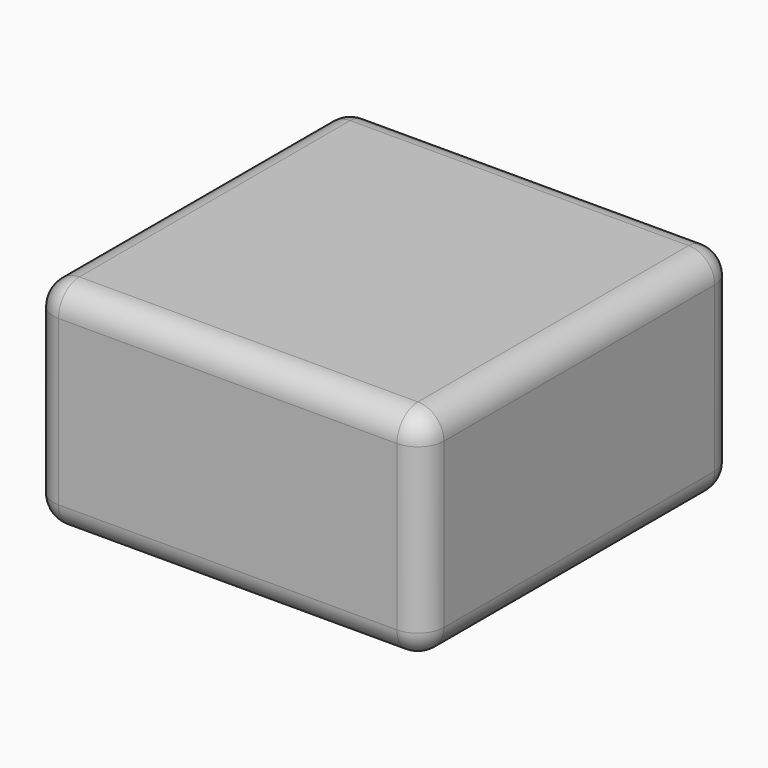
from build123d import *

# Parameters (mm, degrees)
F0_W         = 76.2
F0_H         = 76.2
F0_W_2       = 3.4224579499
F0_H_2       = 7.5862997554
F1_DEPTH     = 42.164
F2_R         = 5.08
F3_T1_DEPTH  = 32.004
F3_S5_W      = 5.08
F3_S5_H      = 5.08
F3_T6_DEPTH  = 5.08
F3_S11_W     = 5.08
F3_S11_H     = 5.08
F3_T12_DEPTH = 5.08


# Not quite as in the source:
# - a fillet or chamfer that OpenCascade refuses, or shapes differently, is made with other operations: its cross-section is extruded or revolved along the edge and cut away or added


with BuildPart() as f1:
    # F0 (on Top) → F1 (new body)
    with BuildSketch(Plane.XY):
        with Locations((-41.3324069232, -13.9183843632)):
            Rectangle(F0_W, F0_H)
        with Locations((-63.0685785115, -38.5174307738)):
            Rectangle(F0_W_2, F0_H_2, mode=Mode.SUBTRACT)
        with Locations((-63.0685785115, -38.5174307738)):
            Rectangle(F0_W_2, F0_H_2)
    extrude(amount=F1_DEPTH)

    # F2
    f2_edges = [f1.edges().sort_by_distance(p)[0] for p in [
        (-41.332407, -52.018384, 0),
        (-3.232407, -13.918384, 0),
        (-41.332407, 24.181616, 0),
        (-79.432407, -13.918384, 0),
        (-79.432407, 24.181616, 21.082),
        (-79.432407, -52.018384, 21.082),
        (-79.432407, -13.918384, 42.164),
        (-41.332407, -52.018384, 42.164),
        (-3.232407, -13.918384, 42.164),
        (-41.332407, 24.181616, 42.164),
        (-3.232407, 24.181616, 21.082),
    ]]
    fillet(f2_edges, radius=F2_R)

    # F3: fillet of radius 5.08 on 1 edges, made by hand

    # F3_s2 → F3_t1 (cut)
    with BuildSketch(Plane.XY.offset(5.08)):
        with BuildLine():
            ThreePointArc((-8.3124069232, -52.0183843632), (-4.7203044747, -50.5304868116), (-3.2324069232, -46.9383843632))
            Line((-3.2324069232, -46.9383843632), (-3.2324069232, -52.0183843632))
            Line((-3.2324069232, -52.0183843632), (-8.3124069232, -52.0183843632))
        make_face()
    extrude(amount=F3_T1_DEPTH, mode=Mode.SUBTRACT)


with BuildPart() as f3_tool4:
    # F3_s5 → F3_t6 (new body)
    with BuildSketch(Plane.XZ.offset(46.9383843632)):
        with Locations((-5.7724069232, 2.54)):
            Rectangle(F3_S5_W, F3_S5_H)
    extrude(amount=F3_T6_DEPTH)

    # F3_s7 → F3_t8 (revolve, cut)
    with BuildSketch(Plane(origin=(-8.3124069232, -46.9383843632, 5.08), x_dir=(-0.7071067812, 0, 0.7071067812), z_dir=(0.7071067812, 0, 0.7071067812))):
        with BuildLine():
            ThreePointArc((0, -5.08), (5.08, 0), (0, 5.08))
            Line((0, 5.08), (0, -5.08))
        make_face()
    revolve(axis=Axis((-8.3124069232, -46.9383843632, 5.08), (0, -1, 0)), mode=Mode.SUBTRACT)


with BuildPart() as f1_1:
    add(f1.part)

    # F3_t3: cut F3_tool4
    add(f3_tool4.part, mode=Mode.SUBTRACT)


with BuildPart() as f3_tool10:
    # F3_s11 → F3_t12 (new body)
    with BuildSketch(Plane.XZ.offset(46.9383843632)):
        with Locations((-5.7724069232, 39.624)):
            Rectangle(F3_S11_W, F3_S11_H)
    extrude(amount=F3_T12_DEPTH)

    # F3_s13 → F3_t14 (revolve, cut)
    with BuildSketch(Plane(origin=(-8.3124069232, -46.9383843632, 37.084), x_dir=(-0.7071067812, 0, -0.7071067812), z_dir=(-0.7071067812, 0, 0.7071067812))):
        with BuildLine():
            ThreePointArc((0, -5.08), (5.08, 0), (0, 5.08))
            Line((0, 5.08), (0, -5.08))
        make_face()
    revolve(axis=Axis((-8.3124069232, -46.9383843632, 37.084), (0, -1, 0)), mode=Mode.SUBTRACT)


with BuildPart() as f1_2:
    add(f1_1.part)

    # F3_t9: cut F3_tool10
    add(f3_tool10.part, mode=Mode.SUBTRACT)


solid = f1_2.part
